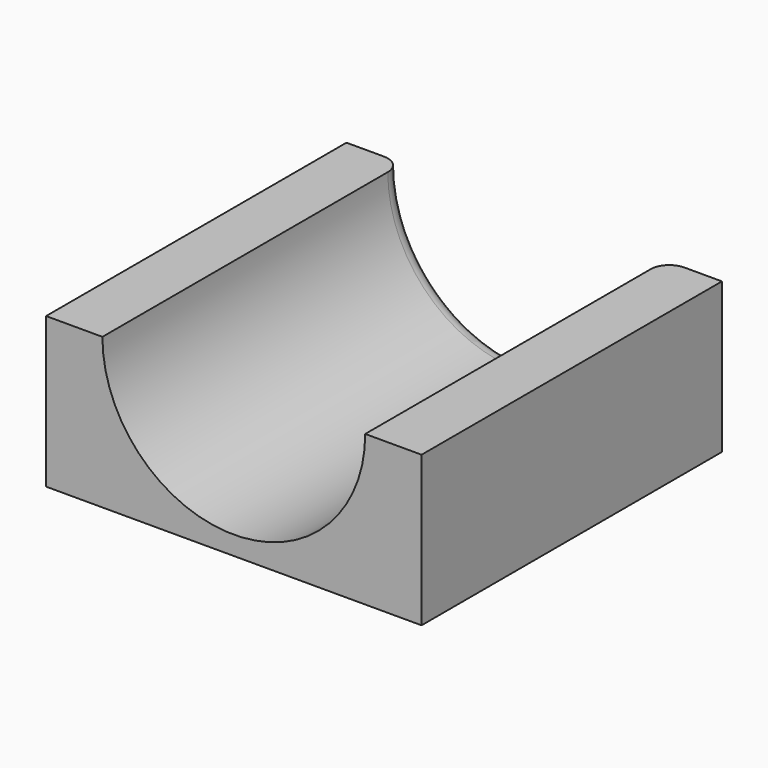
from build123d import *

# Parameters (mm, degrees)
F1_DEPTH = 50
F2_R     = 4.99999


# Not quite as in the source:
# - a fillet or chamfer is up to 0.001 mm smaller than in the source, because OpenCascade refuses the exact size


with BuildPart() as f1:
    # F0 (on Front) → F1 (new body, symmetric)
    with BuildSketch(Plane.XZ):
        with BuildLine():
            Line((-50, 40), (-50, 0))
            Line((-50, 0), (0, 0))
            Line((0, 0), (50, 0))
            Line((50, 0), (50, 40))
            Line((50, 40), (35, 40))
            ThreePointArc((35, 40), (0, 5), (-35, 40))
            Line((-35, 40), (-50, 40))
        make_face()
    extrude(amount=F1_DEPTH, both=True)

    # F2 (radius 5 in the source; OpenCascade refuses exactly that, so slightly less here)
    f2_edges = [f1.edges().sort_by_distance(p)[0] for p in [
        (0, 50, 5),
    ]]
    fillet(f2_edges, radius=F2_R)


solid = f1.part
